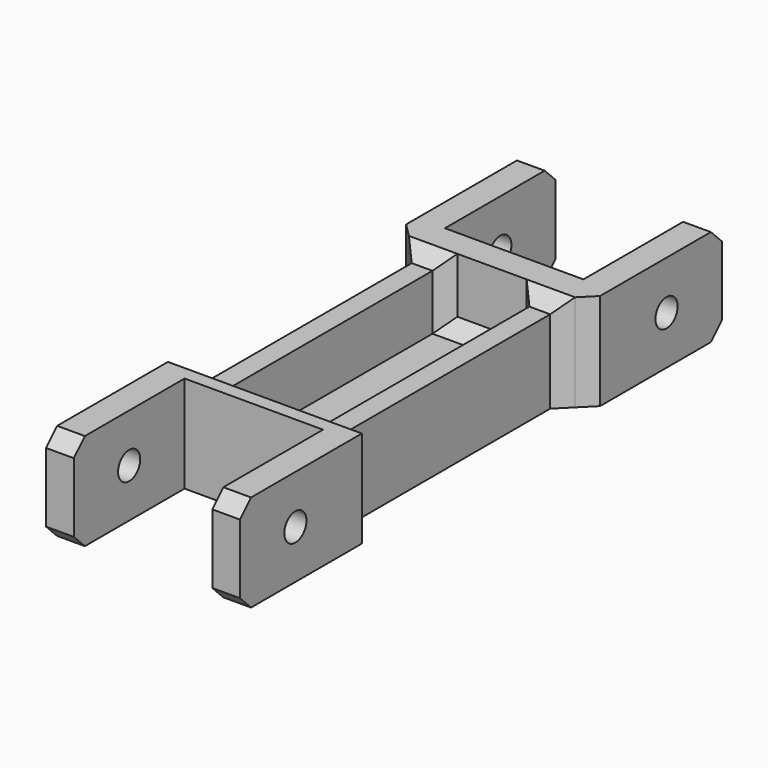
from build123d import *

# Parameters (mm, degrees)
F0_W            = 20
F0_H            = 22
F0_H_2          = 4
F0_H_3          = 20.4
F1_DEPTH        = 2
F2_DEPTH        = 10
F3_R            = 2.2
F4_DEPTH        = 30
F5_W            = 20
F5_H            = 12
F5_R            = 2.6
F7_DEPTH        = 4
F6_W            = 20
F6_H            = 12
F6_R            = 2.6
F8_DEPTH        = 4
F9_T1_DEPTH     = 25
F9_T3_DEPTH     = 57.4
F9_T5_DEPTH     = 16
F9_T7_DEPTH     = 48.4
F9_T9_DEPTH     = 2
F9_T11_DEPTH    = 20
F9_T13_DEPTH    = 7
F9_T15_DEPTH    = 25
F9_T17_DEPTH    = 14
F9_T19_DEPTH    = 27
F9_T21_DEPTH    = 14
F9_T23_DEPTH    = 30
F9_T25_DEPTH    = 7
F9_T27_DEPTH    = 8
F9_S31_W        = 2
F9_S31_H        = 2
F9_T32_DEPTH    = 2
F9_S37_W        = 2
F9_S37_H        = 2
F9_T38_DEPTH    = 2
F9_S43_W        = 2
F9_S43_H        = 2
F9_T44_DEPTH    = 2
F9_S49_W        = 2
F9_S49_H        = 2
F9_T50_DEPTH    = 2
F9_S55_W        = 2
F9_S55_H        = 2
F9_T56_DEPTH    = 2
F9_S61_W        = 2
F9_S61_H        = 2
F9_T62_DEPTH    = 2
F9_S67_W        = 2
F9_S67_H        = 2
F9_T68_DEPTH    = 2
F9_S73_W        = 2
F9_S73_H        = 2
F9_T74_DEPTH    = 2
F9_T81_DEPTH    = 30
F9_T85_DEPTH    = 30
F9_T92_DEPTH    = 7
F9_T96_DEPTH    = 53.4
F9_T103_DEPTH   = 30
F9_T107_DEPTH   = 30
F9_S1_T1_DEPTH  = 7
F9_S1_T3_DEPTH  = 30
F9_S1_T5_DEPTH  = 16
F9_S1_T7_DEPTH  = 8
F9_S1_S11_W     = 2
F9_S1_S11_H     = 2
F9_S1_T12_DEPTH = 2
F9_S1_S17_W     = 2
F9_S1_S17_H     = 2
F9_S1_T18_DEPTH = 2
F9_S1_S23_W     = 2
F9_S1_S23_H     = 2
F9_S1_T24_DEPTH = 2
F9_S1_S29_W     = 2
F9_S1_S29_H     = 2
F9_S1_T30_DEPTH = 2
F10_W           = 20
F10_H           = 47
F11_DEPTH       = 4
F12_W           = 20
F12_H           = 4
F13_DEPTH       = 10
F16_DEPTH       = 4
F17_DEPTH       = 4
F19_W           = 4
F19_H           = 14
F20_DEPTH       = 20
F18_W           = 4
F18_H           = 14
F21_DEPTH       = 20
F22_W           = 39
F22_H           = 8
F23_DEPTH       = 3
F24_W           = 39
F24_H           = 8
F25_DEPTH       = 3
F26_R           = 2
F27_R           = 2
F28_DEPTH       = 28.3421242009
F29_SIZE        = 1.99999


# Not quite as in the source:
# - a fillet or chamfer that OpenCascade refuses, or shapes differently, is made with other operations: its cross-section is extruded or revolved along the edge and cut away or added
# - a fillet or chamfer is up to 0.001 mm smaller than in the source, because OpenCascade refuses the exact size
# - a feature names something its author has since deleted; it is built from what else it names


with BuildPart() as f1:
    # F0 (on Top) → F1 (new body)
    with BuildSketch(Plane.XY):
        with Locations((-44.4073281825, 48.6883277684)):
            Rectangle(F0_W, F0_H)
        with Locations((-44.4073281825, 61.6883277684)):
            Rectangle(F0_W, F0_H_2)
        with Locations((-44.4073281825, 35.6883277684)):
            Rectangle(F0_W, F0_H_2)
        with Locations((-44.4073281825, 23.4883277684)):
            Rectangle(F0_W, F0_H_3)
        with Locations((-44.4073281825, 11.2883277684)):
            Rectangle(F0_W, F0_H_2)
    extrude(amount=-F1_DEPTH)

    # F0 (on Top) → F2 (join)
    with BuildSketch(Plane.XY):
        with Locations((-44.4073281825, 35.6883277684)):
            Rectangle(F0_W, F0_H_2)
        with Locations((-44.4073281825, 61.6883277684)):
            Rectangle(F0_W, F0_H_2)
        with Locations((-44.4073281825, 11.2883277684)):
            Rectangle(F0_W, F0_H_2)
    extrude(amount=F2_DEPTH)

    # F3 (on face) → F4 (cut)
    with BuildSketch(Plane.XZ.offset(-9.2883277684)):
        with Locations((-44.4073281825, 5.5)):
            Circle(F3_R)
    extrude(amount=-F4_DEPTH, mode=Mode.SUBTRACT)

    # F5 (on face) → F7 (join)
    with BuildSketch(Plane(origin=(-54.4073281825, 0, 0), x_dir=(0, -1, 0), z_dir=(-1, 0, 0))):
        with Locations((-73.6883277684, 4)):
            Rectangle(F5_W, F5_H)
        with Locations((-73.6883277684, 4)):
            Circle(F5_R, mode=Mode.SUBTRACT)
    extrude(amount=F7_DEPTH)

    # F6 (on face) → F8 (join)
    with BuildSketch(Plane.YZ.offset(-34.4073281825)):
        with Locations((73.6883277684, 4)):
            Rectangle(F6_W, F6_H)
        with Locations((73.6883277684, 4)):
            Circle(F6_R, mode=Mode.SUBTRACT)
        Polygon((63.6883277684, 10), (59.6883277684, 10), (59.6883277684, 0), (59.6883277684, -2), (63.6883277684, -2), align=None)
    extrude(amount=F8_DEPTH)

    # F9: fillet of radius 2 on 26 edges, made by hand

    # F9_s2 → F9_t1 (cut)
    with BuildSketch(Plane.YZ.offset(-59.4073281825)):
        with BuildLine():
            ThreePointArc((63.6883277684, 0), (63.1025413308, -1.4142135624), (61.6883277684, -2))
            Line((61.6883277684, -2), (63.6883277684, -2))
            Line((63.6883277684, -2), (63.6883277684, 0))
        make_face()
        with BuildLine():
            ThreePointArc((63.6883277684, 8), (63.1025413308, 9.4142135624), (61.6883277684, 10))
            Line((61.6883277684, 10), (63.6883277684, 10))
            Line((63.6883277684, 10), (63.6883277684, 8))
        make_face()
    extrude(amount=F9_T1_DEPTH, mode=Mode.SUBTRACT)

    # F9_s4 → F9_t3 (cut)
    with BuildSketch(Plane.XZ.offset(-68.6883277684)):
        with BuildLine():
            ThreePointArc((-54.4073281825, 0), (-53.8215417448, -1.4142135624), (-52.4073281825, -2))
            Line((-52.4073281825, -2), (-54.4073281825, -2))
            Line((-54.4073281825, -2), (-54.4073281825, 0))
        make_face()
    extrude(amount=F9_T3_DEPTH, mode=Mode.SUBTRACT)

    # F9_s6 → F9_t5 (cut)
    with BuildSketch(Plane.YZ.offset(-52.4073281825)):
        with BuildLine():
            ThreePointArc((9.2883277684, 0), (9.8741142061, -1.4142135624), (11.2883277684, -2))
            Line((11.2883277684, -2), (9.2883277684, -2))
            Line((9.2883277684, -2), (9.2883277684, 0))
        make_face()
        with BuildLine():
            ThreePointArc((9.2883277684, 8), (9.8741142061, 9.4142135624), (11.2883277684, 10))
            Line((11.2883277684, 10), (9.2883277684, 10))
            Line((9.2883277684, 10), (9.2883277684, 8))
        make_face()
    extrude(amount=F9_T5_DEPTH, mode=Mode.SUBTRACT)

    # F9_s8 → F9_t7 (cut)
    with BuildSketch(Plane.XZ.offset(-59.6883277684)):
        with BuildLine():
            ThreePointArc((-34.4073281825, 0), (-34.9931146201, -1.4142135624), (-36.4073281825, -2))
            Line((-36.4073281825, -2), (-34.4073281825, -2))
            Line((-34.4073281825, -2), (-34.4073281825, 0))
        make_face()
    extrude(amount=F9_T7_DEPTH, mode=Mode.SUBTRACT)

    # F9_s10 → F9_t9 (cut)
    with BuildSketch(Plane.YZ.offset(-34.4073281825)):
        with BuildLine():
            ThreePointArc((59.6883277684, 0), (60.2741142061, -1.4142135624), (61.6883277684, -2))
            Line((61.6883277684, -2), (59.6883277684, -2))
            Line((59.6883277684, -2), (59.6883277684, 0))
        make_face()
    extrude(amount=F9_T9_DEPTH, mode=Mode.SUBTRACT)

    # F9_s12 → F9_t11 (cut)
    with BuildSketch(Plane.XZ.offset(-81.6883277684)):
        with BuildLine():
            ThreePointArc((-30.4073281825, 0), (-30.9931146201, -1.4142135624), (-32.4073281825, -2))
            Line((-32.4073281825, -2), (-30.4073281825, -2))
            Line((-30.4073281825, -2), (-30.4073281825, 0))
        make_face()
        with BuildLine():
            ThreePointArc((-30.4073281825, 8), (-30.9931146201, 9.4142135624), (-32.4073281825, 10))
            Line((-32.4073281825, 10), (-30.4073281825, 10))
            Line((-30.4073281825, 10), (-30.4073281825, 8))
        make_face()
    extrude(amount=F9_T11_DEPTH, mode=Mode.SUBTRACT)

    # F9_s14 → F9_t13 (cut)
    with BuildSketch(Plane.YZ.offset(-39.4073281825)):
        with BuildLine():
            ThreePointArc((83.6883277684, 0), (83.1025413308, -1.4142135624), (81.6883277684, -2))
            Line((81.6883277684, -2), (83.6883277684, -2))
            Line((83.6883277684, -2), (83.6883277684, 0))
        make_face()
        with BuildLine():
            ThreePointArc((83.6883277684, 8), (83.1025413308, 9.4142135624), (81.6883277684, 10))
            Line((81.6883277684, 10), (83.6883277684, 10))
            Line((83.6883277684, 10), (83.6883277684, 8))
        make_face()
    extrude(amount=F9_T13_DEPTH, mode=Mode.SUBTRACT)

    # F9_s16 → F9_t15 (cut)
    with BuildSketch(Plane.XZ.offset(-88.6883277684)):
        with BuildLine():
            ThreePointArc((-34.4073281825, 0), (-33.8215417448, -1.4142135624), (-32.4073281825, -2))
            Line((-32.4073281825, -2), (-34.4073281825, -2))
            Line((-34.4073281825, -2), (-34.4073281825, 0))
        make_face()
        with BuildLine():
            ThreePointArc((-34.4073281825, 8), (-33.8215417448, 9.4142135624), (-32.4073281825, 10))
            Line((-32.4073281825, 10), (-34.4073281825, 10))
            Line((-34.4073281825, 10), (-34.4073281825, 8))
        make_face()
    extrude(amount=F9_T15_DEPTH, mode=Mode.SUBTRACT)

    # F9_s18 → F9_t17 (cut)
    with BuildSketch(Plane.XZ.offset(-68.6883277684)):
        with BuildLine():
            ThreePointArc((-52.4073281825, 10), (-53.8215417448, 9.4142135624), (-54.4073281825, 8))
            Line((-54.4073281825, 8), (-54.4073281825, 10))
            Line((-54.4073281825, 10), (-52.4073281825, 10))
        make_face()
    extrude(amount=F9_T17_DEPTH, mode=Mode.SUBTRACT)

    # F9_s20 → F9_t19 (cut)
    with BuildSketch(Plane.YZ.offset(-59.4073281825)):
        with BuildLine():
            ThreePointArc((59.6883277684, 8), (60.2741142061, 9.4142135624), (61.6883277684, 10))
            Line((61.6883277684, 10), (59.6883277684, 10))
            Line((59.6883277684, 10), (59.6883277684, 8))
        make_face()
    extrude(amount=F9_T19_DEPTH, mode=Mode.SUBTRACT)

    # F9_s22 → F9_t21 (cut)
    with BuildSketch(Plane.XZ.offset(-42.6883277684)):
        with BuildLine():
            ThreePointArc((-52.4073281825, 10), (-53.8215417448, 9.4142135624), (-54.4073281825, 8))
            Line((-54.4073281825, 8), (-54.4073281825, 10))
            Line((-54.4073281825, 10), (-52.4073281825, 10))
        make_face()
        with BuildLine():
            ThreePointArc((-36.4073281825, 10), (-34.9931146201, 9.4142135624), (-34.4073281825, 8))
            Line((-34.4073281825, 8), (-34.4073281825, 10))
            Line((-34.4073281825, 10), (-36.4073281825, 10))
        make_face()
    extrude(amount=F9_T21_DEPTH, mode=Mode.SUBTRACT)

    # F9_s24 → F9_t23 (cut)
    with BuildSketch(Plane.YZ.offset(-59.4073281825)):
        with BuildLine():
            ThreePointArc((33.6883277684, 8), (34.2741142061, 9.4142135624), (35.6883277684, 10))
            Line((35.6883277684, 10), (33.6883277684, 10))
            Line((33.6883277684, 10), (33.6883277684, 8))
        make_face()
        with BuildLine():
            ThreePointArc((37.6883277684, 8), (37.1025413308, 9.4142135624), (35.6883277684, 10))
            Line((35.6883277684, 10), (37.6883277684, 10))
            Line((37.6883277684, 10), (37.6883277684, 8))
        make_face()
        with BuildLine():
            ThreePointArc((13.2883277684, 8), (12.7025413308, 9.4142135624), (11.2883277684, 10))
            Line((11.2883277684, 10), (13.2883277684, 10))
            Line((13.2883277684, 10), (13.2883277684, 8))
        make_face()
    extrude(amount=F9_T23_DEPTH, mode=Mode.SUBTRACT)

    # F9_s26 → F9_t25 (cut)
    with BuildSketch(Plane.XZ.offset(-18.2883277684)):
        with BuildLine():
            ThreePointArc((-36.4073281825, 10), (-34.9931146201, 9.4142135624), (-34.4073281825, 8))
            Line((-34.4073281825, 8), (-34.4073281825, 10))
            Line((-34.4073281825, 10), (-36.4073281825, 10))
        make_face()
        with BuildLine():
            ThreePointArc((-52.4073281825, 10), (-53.8215417448, 9.4142135624), (-54.4073281825, 8))
            Line((-54.4073281825, 8), (-54.4073281825, 10))
            Line((-54.4073281825, 10), (-52.4073281825, 10))
        make_face()
    extrude(amount=F9_T25_DEPTH, mode=Mode.SUBTRACT)

    # F9_s28 → F9_t27 (cut)
    with BuildSketch(Plane.XY):
        with BuildLine():
            ThreePointArc((-36.4073281825, 9.2883277684), (-34.9931146201, 9.8741142061), (-34.4073281825, 11.2883277684))
            Line((-34.4073281825, 11.2883277684), (-34.4073281825, 9.2883277684))
            Line((-34.4073281825, 9.2883277684), (-36.4073281825, 9.2883277684))
        make_face()
        with BuildLine():
            ThreePointArc((-52.4073281825, 9.2883277684), (-53.8215417448, 9.8741142061), (-54.4073281825, 11.2883277684))
            Line((-54.4073281825, 11.2883277684), (-54.4073281825, 9.2883277684))
            Line((-54.4073281825, 9.2883277684), (-52.4073281825, 9.2883277684))
        make_face()
        with BuildLine():
            ThreePointArc((-30.4073281825, 61.6883277684), (-30.9931146201, 60.2741142061), (-32.4073281825, 59.6883277684))
            Line((-32.4073281825, 59.6883277684), (-30.4073281825, 59.6883277684))
            Line((-30.4073281825, 59.6883277684), (-30.4073281825, 61.6883277684))
        make_face()
        with BuildLine():
            ThreePointArc((-30.4073281825, 81.6883277684), (-30.9931146201, 83.1025413308), (-32.4073281825, 83.6883277684))
            Line((-32.4073281825, 83.6883277684), (-30.4073281825, 83.6883277684))
            Line((-30.4073281825, 83.6883277684), (-30.4073281825, 81.6883277684))
        make_face()
    extrude(amount=F9_T27_DEPTH, mode=Mode.SUBTRACT)


with BuildPart() as f9_tool30:
    # F9_s31 → F9_t32 (new body)
    with BuildSketch(Plane.YZ.offset(-52.4073281825)):
        with Locations((10.2883277684, -1)):
            Rectangle(F9_S31_W, F9_S31_H)
    extrude(amount=-F9_T32_DEPTH)

    # F9_s33 → F9_t34 (revolve, cut)
    with BuildSketch(Plane(origin=(-52.4073281825, 11.2883277684, 0), x_dir=(0, 0.7071067812, 0.7071067812), z_dir=(0, -0.7071067812, 0.7071067812))):
        with BuildLine():
            ThreePointArc((0, -2), (2, 0), (0, 2))
            Line((0, 2), (0, -2))
        make_face()
    revolve(axis=Axis((-52.4073281825, 11.2883277684, 0), (-1, 0, 0)), mode=Mode.SUBTRACT)


with BuildPart() as f1_1:
    add(f1.part)

    # F9_t29: cut F9_tool30
    add(f9_tool30.part, mode=Mode.SUBTRACT)


with BuildPart() as f9_tool36:
    # F9_s37 → F9_t38 (new body)
    with BuildSketch(Plane.XY):
        with Locations((-35.4073281825, 10.2883277684)):
            Rectangle(F9_S37_W, F9_S37_H)
    extrude(amount=-F9_T38_DEPTH)

    # F9_s39 → F9_t40 (revolve, cut)
    with BuildSketch(Plane(origin=(-36.4073281825, 11.2883277684, 0), x_dir=(-0.7071067812, 0.7071067812, 0), z_dir=(-0.7071067812, -0.7071067812, 0))):
        with BuildLine():
            ThreePointArc((0, -2), (2, 0), (0, 2))
            Line((0, 2), (0, -2))
        make_face()
    revolve(axis=Axis((-36.4073281825, 11.2883277684, 0), (0, 0, -1)), mode=Mode.SUBTRACT)


with BuildPart() as f1_2:
    add(f1_1.part)

    # F9_t35: cut F9_tool36
    add(f9_tool36.part, mode=Mode.SUBTRACT)


with BuildPart() as f9_tool42:
    # F9_s43 → F9_t44 (new body)
    with BuildSketch(Plane.YZ.offset(-32.4073281825)):
        with Locations((60.6883277684, -1)):
            Rectangle(F9_S43_W, F9_S43_H)
    extrude(amount=F9_T44_DEPTH)

    # F9_s45 → F9_t46 (revolve, cut)
    with BuildSketch(Plane(origin=(-32.4073281825, 61.6883277684, 0), x_dir=(0, 0.7071067812, 0.7071067812), z_dir=(0, 0.7071067812, -0.7071067812))):
        with BuildLine():
            ThreePointArc((0, -2), (2, 0), (0, 2))
            Line((0, 2), (0, -2))
        make_face()
    revolve(axis=Axis((-32.4073281825, 61.6883277684, 0), (1, 0, 0)), mode=Mode.SUBTRACT)


with BuildPart() as f1_3:
    add(f1_2.part)

    # F9_t41: cut F9_tool42
    add(f9_tool42.part, mode=Mode.SUBTRACT)


with BuildPart() as f9_tool48:
    # F9_s49 → F9_t50 (new body)
    with BuildSketch(Plane.XY):
        with Locations((-31.4073281825, 82.6883277684)):
            Rectangle(F9_S49_W, F9_S49_H)
    extrude(amount=-F9_T50_DEPTH)

    # F9_s51 → F9_t52 (revolve, cut)
    with BuildSketch(Plane(origin=(-32.4073281825, 81.6883277684, 0), x_dir=(-0.7071067812, -0.7071067812, 0), z_dir=(0.7071067812, -0.7071067812, 0))):
        with BuildLine():
            ThreePointArc((0, -2), (2, 0), (0, 2))
            Line((0, 2), (0, -2))
        make_face()
    revolve(axis=Axis((-32.4073281825, 81.6883277684, 0), (0, 0, -1)), mode=Mode.SUBTRACT)


with BuildPart() as f1_4:
    add(f1_3.part)

    # F9_t47: cut F9_tool48
    add(f9_tool48.part, mode=Mode.SUBTRACT)


with BuildPart() as f9_tool54:
    # F9_s55 → F9_t56 (new body)
    with BuildSketch(Plane.XY.offset(8)):
        with Locations((-31.4073281825, 60.6883277684)):
            Rectangle(F9_S55_W, F9_S55_H)
    extrude(amount=F9_T56_DEPTH)

    # F9_s57 → F9_t58 (revolve, cut)
    with BuildSketch(Plane(origin=(-32.4073281825, 61.6883277684, 8), x_dir=(-0.7071067812, 0.7071067812, 0), z_dir=(0.7071067812, 0.7071067812, 0))):
        with BuildLine():
            ThreePointArc((0, -2), (2, 0), (0, 2))
            Line((0, 2), (0, -2))
        make_face()
    revolve(axis=Axis((-32.4073281825, 61.6883277684, 8), (0, 0, 1)), mode=Mode.SUBTRACT)


with BuildPart() as f1_5:
    add(f1_4.part)

    # F9_t53: cut F9_tool54
    add(f9_tool54.part, mode=Mode.SUBTRACT)


with BuildPart() as f9_tool60:
    # F9_s61 → F9_t62 (new body)
    with BuildSketch(Plane.XZ.offset(-81.6883277684)):
        with Locations((-31.4073281825, 9)):
            Rectangle(F9_S61_W, F9_S61_H)
    extrude(amount=-F9_T62_DEPTH)

    # F9_s63 → F9_t64 (revolve, cut)
    with BuildSketch(Plane(origin=(-32.4073281825, 81.6883277684, 8), x_dir=(-0.7071067812, 0, -0.7071067812), z_dir=(0.7071067812, 0, -0.7071067812))):
        with BuildLine():
            ThreePointArc((0, -2), (2, 0), (0, 2))
            Line((0, 2), (0, -2))
        make_face()
    revolve(axis=Axis((-32.4073281825, 81.6883277684, 8), (0, 1, 0)), mode=Mode.SUBTRACT)


with BuildPart() as f1_6:
    add(f1_5.part)

    # F9_t59: cut F9_tool60
    add(f9_tool60.part, mode=Mode.SUBTRACT)


with BuildPart() as f9_tool66:
    # F9_s67 → F9_t68 (new body)
    with BuildSketch(Plane.XZ.offset(-11.2883277684)):
        with Locations((-35.4073281825, 9)):
            Rectangle(F9_S67_W, F9_S67_H)
    extrude(amount=F9_T68_DEPTH)

    # F9_s69 → F9_t70 (revolve, cut)
    with BuildSketch(Plane(origin=(-36.4073281825, 11.2883277684, 8), x_dir=(-0.7071067812, 0, -0.7071067812), z_dir=(-0.7071067812, 0, 0.7071067812))):
        with BuildLine():
            ThreePointArc((0, -2), (2, 0), (0, 2))
            Line((0, 2), (0, -2))
        make_face()
    revolve(axis=Axis((-36.4073281825, 11.2883277684, 8), (0, -1, 0)), mode=Mode.SUBTRACT)


with BuildPart() as f1_7:
    add(f1_6.part)

    # F9_t65: cut F9_tool66
    add(f9_tool66.part, mode=Mode.SUBTRACT)


with BuildPart() as f9_tool72:
    # F9_s73 → F9_t74 (new body)
    with BuildSketch(Plane.YZ.offset(-52.4073281825)):
        with Locations((10.2883277684, 9)):
            Rectangle(F9_S73_W, F9_S73_H)
    extrude(amount=-F9_T74_DEPTH)

    # F9_s75 → F9_t76 (revolve, cut)
    with BuildSketch(Plane(origin=(-52.4073281825, 11.2883277684, 8), x_dir=(0, 0.7071067812, -0.7071067812), z_dir=(0, 0.7071067812, 0.7071067812))):
        with BuildLine():
            ThreePointArc((0, -2), (2, 0), (0, 2))
            Line((0, 2), (0, -2))
        make_face()
    revolve(axis=Axis((-52.4073281825, 11.2883277684, 8), (-1, 0, 0)), mode=Mode.SUBTRACT)


with BuildPart() as f1_8:
    add(f1_7.part)

    # F9_t71: cut F9_tool72
    add(f9_tool72.part, mode=Mode.SUBTRACT)


with BuildPart() as f9_tool79:
    # F9_s80 → F9_t81 (new body)
    with BuildSketch(Plane.YZ.offset(-29.4073281825)):
        with BuildLine():
            ThreePointArc((63.6883277684, 0), (63.1025413308, -1.4142135624), (61.6883277684, -2))
            Line((61.6883277684, -2), (63.6883277684, -2))
            Line((63.6883277684, -2), (63.6883277684, 0))
        make_face()
    extrude(amount=-F9_T81_DEPTH)

    split(bisect_by=Plane.YZ.offset(-34.4073281825), keep=Keep.TOP)


with BuildPart() as f9_tool83:
    # F9_s84 → F9_t85 (new body)
    with BuildSketch(Plane.XZ.offset(-58.6883277684)):
        with BuildLine():
            ThreePointArc((-34.4073281825, 0), (-33.8215417448, -1.4142135624), (-32.4073281825, -2))
            Line((-32.4073281825, -2), (-34.4073281825, -2))
            Line((-34.4073281825, -2), (-34.4073281825, 0))
        make_face()
    extrude(amount=-F9_T85_DEPTH)

    split(bisect_by=Plane.XZ.offset(-63.6883277684), keep=Keep.TOP)


with BuildPart() as f9_tool79_1:
    add(f9_tool79.part)

    # F9_t87: intersect F9_tool83
    add(f9_tool83.part, mode=Mode.INTERSECT)


with BuildPart() as f1_9:
    add(f1_8.part)

    # F9_t77: cut F9_tool79
    add(f9_tool79_1.part, mode=Mode.SUBTRACT)


with BuildPart() as f9_tool90:
    # F9_s91 → F9_t92 (new body)
    with BuildSketch(Plane.YZ.offset(-39.4073281825)):
        with BuildLine():
            ThreePointArc((59.6883277684, 0), (60.2741142061, -1.4142135624), (61.6883277684, -2))
            Line((61.6883277684, -2), (59.6883277684, -2))
            Line((59.6883277684, -2), (59.6883277684, 0))
        make_face()
    extrude(amount=F9_T92_DEPTH)

    split(bisect_by=Plane.YZ.offset(-34.4073281825), keep=Keep.BOTTOM)


with BuildPart() as f9_tool94:
    # F9_s95 → F9_t96 (new body)
    with BuildSketch(Plane.XZ.offset(-11.2883277684)):
        with BuildLine():
            ThreePointArc((-34.4073281825, 0), (-34.9931146201, -1.4142135624), (-36.4073281825, -2))
            Line((-36.4073281825, -2), (-34.4073281825, -2))
            Line((-34.4073281825, -2), (-34.4073281825, 0))
        make_face()
    extrude(amount=-F9_T96_DEPTH)

    split(bisect_by=Plane.XZ.offset(-59.6883277684), keep=Keep.BOTTOM)


with BuildPart() as f9_tool90_1:
    add(f9_tool90.part)

    # F9_t98: intersect F9_tool94
    add(f9_tool94.part, mode=Mode.INTERSECT)


with BuildPart() as f1_10:
    add(f1_9.part)

    # F9_t88: cut F9_tool90
    add(f9_tool90_1.part, mode=Mode.SUBTRACT)


with BuildPart() as f9_tool101:
    # F9_s102 → F9_t103 (new body)
    with BuildSketch(Plane.YZ.offset(-29.4073281825)):
        with BuildLine():
            ThreePointArc((63.6883277684, 8), (63.1025413308, 9.4142135624), (61.6883277684, 10))
            Line((61.6883277684, 10), (63.6883277684, 10))
            Line((63.6883277684, 10), (63.6883277684, 8))
        make_face()
    extrude(amount=-F9_T103_DEPTH)

    split(bisect_by=Plane.YZ.offset(-34.4073281825), keep=Keep.TOP)


with BuildPart() as f9_tool105:
    # F9_s106 → F9_t107 (new body)
    with BuildSketch(Plane.XZ.offset(-88.6883277684)):
        with BuildLine():
            ThreePointArc((-34.4073281825, 8), (-33.8215417448, 9.4142135624), (-32.4073281825, 10))
            Line((-32.4073281825, 10), (-34.4073281825, 10))
            Line((-34.4073281825, 10), (-34.4073281825, 8))
        make_face()
    extrude(amount=F9_T107_DEPTH)

    split(bisect_by=Plane.XZ.offset(-63.6883277684), keep=Keep.TOP)


with BuildPart() as f9_tool101_1:
    add(f9_tool101.part)

    # F9_t109: intersect F9_tool105
    add(f9_tool105.part, mode=Mode.INTERSECT)


with BuildPart() as f1_11:
    add(f1_10.part)

    # F9_t99: cut F9_tool101
    add(f9_tool101_1.part, mode=Mode.SUBTRACT)

    # F9#s1: fillet of radius 2 on 10 edges, made by hand

    # F9_s1_s2 → F9_s1_t1 (cut)
    with BuildSketch(Plane.YZ.offset(-56.4073281825)):
        with BuildLine():
            ThreePointArc((83.6883277684, 0), (83.1025413308, -1.4142135624), (81.6883277684, -2))
            Line((81.6883277684, -2), (83.6883277684, -2))
            Line((83.6883277684, -2), (83.6883277684, 0))
        make_face()
        with BuildLine():
            ThreePointArc((63.6883277684, 0), (64.2741142061, -1.4142135624), (65.6883277684, -2))
            Line((65.6883277684, -2), (63.6883277684, -2))
            Line((63.6883277684, -2), (63.6883277684, 0))
        make_face()
        with BuildLine():
            ThreePointArc((63.6883277684, 8), (64.2741142061, 9.4142135624), (65.6883277684, 10))
            Line((65.6883277684, 10), (63.6883277684, 10))
            Line((63.6883277684, 10), (63.6883277684, 8))
        make_face()
        with BuildLine():
            ThreePointArc((81.6883277684, 10), (83.1025413308, 9.4142135624), (83.6883277684, 8))
            Line((83.6883277684, 8), (83.6883277684, 10))
            Line((83.6883277684, 10), (81.6883277684, 10))
        make_face()
    extrude(amount=F9_S1_T1_DEPTH, mode=Mode.SUBTRACT)

    # F9_s1_s4 → F9_s1_t3 (cut)
    with BuildSketch(Plane.XZ.offset(-88.6883277684)):
        with BuildLine():
            ThreePointArc((-56.4073281825, -2), (-54.9931146201, -1.4142135624), (-54.4073281825, 0))
            Line((-54.4073281825, 0), (-54.4073281825, -2))
            Line((-54.4073281825, -2), (-56.4073281825, -2))
        make_face()
        with BuildLine():
            ThreePointArc((-56.4073281825, 10), (-54.9931146201, 9.4142135624), (-54.4073281825, 8))
            Line((-54.4073281825, 8), (-54.4073281825, 10))
            Line((-54.4073281825, 10), (-56.4073281825, 10))
        make_face()
    extrude(amount=F9_S1_T3_DEPTH, mode=Mode.SUBTRACT)

    # F9_s1_s6 → F9_s1_t5 (cut)
    with BuildSketch(Plane.XZ.offset(-81.6883277684)):
        with BuildLine():
            ThreePointArc((-58.4073281825, 0), (-57.8215417448, -1.4142135624), (-56.4073281825, -2))
            Line((-56.4073281825, -2), (-58.4073281825, -2))
            Line((-58.4073281825, -2), (-58.4073281825, 0))
        make_face()
        with BuildLine():
            ThreePointArc((-56.4073281825, 10), (-57.8215417448, 9.4142135624), (-58.4073281825, 8))
            Line((-58.4073281825, 8), (-58.4073281825, 10))
            Line((-58.4073281825, 10), (-56.4073281825, 10))
        make_face()
    extrude(amount=F9_S1_T5_DEPTH, mode=Mode.SUBTRACT)

    # F9_s1_s8 → F9_s1_t7 (cut)
    with BuildSketch(Plane.XY):
        with BuildLine():
            ThreePointArc((-56.4073281825, 63.6883277684), (-57.8215417448, 64.2741142061), (-58.4073281825, 65.6883277684))
            Line((-58.4073281825, 65.6883277684), (-58.4073281825, 63.6883277684))
            Line((-58.4073281825, 63.6883277684), (-56.4073281825, 63.6883277684))
        make_face()
        with BuildLine():
            ThreePointArc((-56.4073281825, 83.6883277684), (-57.8215417448, 83.1025413308), (-58.4073281825, 81.6883277684))
            Line((-58.4073281825, 81.6883277684), (-58.4073281825, 83.6883277684))
            Line((-58.4073281825, 83.6883277684), (-56.4073281825, 83.6883277684))
        make_face()
    extrude(amount=F9_S1_T7_DEPTH, mode=Mode.SUBTRACT)


with BuildPart() as f9_s1_tool10:
    # F9_s1_s11 → F9_s1_t12 (new body)
    with BuildSketch(Plane.XZ.offset(-81.6883277684)):
        with Locations((-57.4073281825, -1)):
            Rectangle(F9_S1_S11_W, F9_S1_S11_H)
    extrude(amount=-F9_S1_T12_DEPTH)

    # F9_s1_s13 → F9_s1_t14 (revolve, cut)
    with BuildSketch(Plane(origin=(-56.4073281825, 81.6883277684, 0), x_dir=(0.7071067812, 0, 0.7071067812), z_dir=(-0.7071067812, 0, 0.7071067812))):
        with BuildLine():
            ThreePointArc((0, -2), (2, 0), (0, 2))
            Line((0, 2), (0, -2))
        make_face()
    revolve(axis=Axis((-56.4073281825, 81.6883277684, 0), (0, 1, 0)), mode=Mode.SUBTRACT)


with BuildPart() as f1_12:
    add(f1_11.part)

    # F9_s1_t9: cut F9_s1_tool10
    add(f9_s1_tool10.part, mode=Mode.SUBTRACT)


with BuildPart() as f9_s1_tool16:
    # F9_s1_s17 → F9_s1_t18 (new body)
    with BuildSketch(Plane.XZ.offset(-65.6883277684)):
        with Locations((-57.4073281825, -1)):
            Rectangle(F9_S1_S17_W, F9_S1_S17_H)
    extrude(amount=F9_S1_T18_DEPTH)

    # F9_s1_s19 → F9_s1_t20 (revolve, cut)
    with BuildSketch(Plane(origin=(-56.4073281825, 65.6883277684, 0), x_dir=(0.7071067812, 0, 0.7071067812), z_dir=(0.7071067812, 0, -0.7071067812))):
        with BuildLine():
            ThreePointArc((0, -2), (2, 0), (0, 2))
            Line((0, 2), (0, -2))
        make_face()
    revolve(axis=Axis((-56.4073281825, 65.6883277684, 0), (0, -1, 0)), mode=Mode.SUBTRACT)


with BuildPart() as f1_13:
    add(f1_12.part)

    # F9_s1_t15: cut F9_s1_tool16
    add(f9_s1_tool16.part, mode=Mode.SUBTRACT)


with BuildPart() as f9_s1_tool22:
    # F9_s1_s23 → F9_s1_t24 (new body)
    with BuildSketch(Plane.XZ.offset(-65.6883277684)):
        with Locations((-57.4073281825, 9)):
            Rectangle(F9_S1_S23_W, F9_S1_S23_H)
    extrude(amount=F9_S1_T24_DEPTH)

    # F9_s1_s25 → F9_s1_t26 (revolve, cut)
    with BuildSketch(Plane(origin=(-56.4073281825, 65.6883277684, 8), x_dir=(0.7071067812, 0, -0.7071067812), z_dir=(-0.7071067812, 0, -0.7071067812))):
        with BuildLine():
            ThreePointArc((0, -2), (2, 0), (0, 2))
            Line((0, 2), (0, -2))
        make_face()
    revolve(axis=Axis((-56.4073281825, 65.6883277684, 8), (0, -1, 0)), mode=Mode.SUBTRACT)


with BuildPart() as f1_14:
    add(f1_13.part)

    # F9_s1_t21: cut F9_s1_tool22
    add(f9_s1_tool22.part, mode=Mode.SUBTRACT)


with BuildPart() as f9_s1_tool28:
    # F9_s1_s29 → F9_s1_t30 (new body)
    with BuildSketch(Plane.XY.offset(8)):
        with Locations((-57.4073281825, 82.6883277684)):
            Rectangle(F9_S1_S29_W, F9_S1_S29_H)
    extrude(amount=F9_S1_T30_DEPTH)

    # F9_s1_s31 → F9_s1_t32 (revolve, cut)
    with BuildSketch(Plane(origin=(-56.4073281825, 81.6883277684, 8), x_dir=(0.7071067812, -0.7071067812, 0), z_dir=(-0.7071067812, -0.7071067812, 0))):
        with BuildLine():
            ThreePointArc((0, -2), (2, 0), (0, 2))
            Line((0, 2), (0, -2))
        make_face()
    revolve(axis=Axis((-56.4073281825, 81.6883277684, 8), (0, 0, 1)), mode=Mode.SUBTRACT)


with BuildPart() as f1_15:
    add(f1_14.part)

    # F9_s1_t27: cut F9_s1_tool28
    add(f9_s1_tool28.part, mode=Mode.SUBTRACT)


with BuildPart() as f11:
    # F10 (on Top) → F11 (new body)
    with BuildSketch(Plane.XY):
        with Locations((-44.0662039816, -58.3389573097)):
            Rectangle(F10_W, F10_H)
    extrude(amount=F11_DEPTH)

    # F12 (on face) → F13 (join)
    with BuildSketch(Plane.XY.offset(4)):
        with Locations((-44.0662039816, -36.8389573097)):
            Rectangle(F12_W, F12_H)
        with Locations((-44.0662039816, -79.8389573097)):
            Rectangle(F12_W, F12_H)
    extrude(amount=F13_DEPTH)

    # F15 (on face) → F16 (join)
    with BuildSketch(Plane.YZ.offset(-34.0662039816)):
        Polygon((-77.8389573097, 0), (-77.8389573097, 4), (-77.8389573097, 14), (-81.8389573097, 14), (-81.8389573097, 0), align=None)
        Polygon((-38.8389573097, 14), (-38.8389573097, 4), (-38.8389573097, 0), (-34.8389573097, 0), (-34.8389573097, 14), align=None)
    extrude(amount=F16_DEPTH)

    # F14 (on face) → F17 (join)
    with BuildSketch(Plane(origin=(-54.0662039816, 0, 0), x_dir=(0, -1, 0), z_dir=(-1, 0, 0))):
        Polygon((38.8389573097, 0), (38.8389573097, 4), (38.8389573097, 14), (34.8389573097, 14), (34.8389573097, 0), align=None)
        Polygon((77.8389573097, 14), (77.8389573097, 4), (77.8389573097, 0), (81.8389573097, 0), (81.8389573097, 14), align=None)
    extrude(amount=F17_DEPTH)

    # F19 (on face) → F20 (join)
    with BuildSketch(Plane.XZ.offset(81.8389573097)):
        with Locations((-56.0662039816, 7)):
            Rectangle(F19_W, F19_H)
        with Locations((-32.0662039816, 7)):
            Rectangle(F19_W, F19_H)
    extrude(amount=F20_DEPTH)

    # F18 (on face) → F21 (join)
    with BuildSketch(Plane(origin=(0, -34.8389573097, 0), x_dir=(-1, 0, 0), z_dir=(0, 1, 0))):
        with Locations((32.0662039816, 7)):
            Rectangle(F18_W, F18_H)
        with Locations((56.0662039816, 7)):
            Rectangle(F18_W, F18_H)
    extrude(amount=F21_DEPTH)

    # F22 (on face) → F23 (join)
    with BuildSketch(Plane(origin=(-54.0662039816, 0, 0), x_dir=(0, -1, 0), z_dir=(-1, 0, 0))):
        with Locations((58.3389573097, 8)):
            Rectangle(F22_W, F22_H)
    extrude(amount=-F23_DEPTH)

    # F24 (on face) → F25 (join)
    with BuildSketch(Plane.YZ.offset(-34.0662039816)):
        with Locations((-58.3389573097, 8)):
            Rectangle(F24_W, F24_H)
    extrude(amount=-F25_DEPTH)

    # F26 (on face) + F27 (on face) → F28 (cut, through all)
    with BuildSketch(Plane.YZ.offset(-30.0662039816)):
        with Locations((-91.8389573097, 7)):
            Circle(F26_R)
    with BuildSketch(Plane.YZ.offset(-30.0662039816)):
        with Locations((-24.8389573097, 7)):
            Circle(F27_R)
    extrude(amount=-F28_DEPTH, mode=Mode.SUBTRACT)

    # F29 (size 2 in the source; OpenCascade refuses exactly that, so slightly less here)
    f29_edges = [f11.edges().sort_by_distance(p)[0] for p in [
        (-32.066204, -101.838957, 0),
        (-30.066204, -77.838957, 7),
        (-44.066204, -77.838957, 4),
        (-44.066204, -77.838957, 14),
        (-58.066204, -77.838957, 7),
        (-44.066204, -38.838957, 4),
        (-51.066204, -38.838957, 8),
        (-37.066204, -38.838957, 8),
        (-34.066204, -38.838957, 6),
        (-35.566204, -38.838957, 12),
        (-52.566204, -38.838957, 12),
        (-54.066204, -38.838957, 6),
        (-30.066204, -38.838957, 7),
        (-58.066204, -38.838957, 7),
        (-32.066204, -14.838957, 14),
        (-56.066204, -14.838957, 14),
        (-56.066204, -14.838957, 0),
        (-32.066204, -14.838957, 0),
        (-56.066204, -101.838957, 14),
        (-32.066204, -101.838957, 14),
        (-56.066204, -101.838957, 0),
    ]]
    chamfer(f29_edges, length=F29_SIZE)


solid = f11.part
